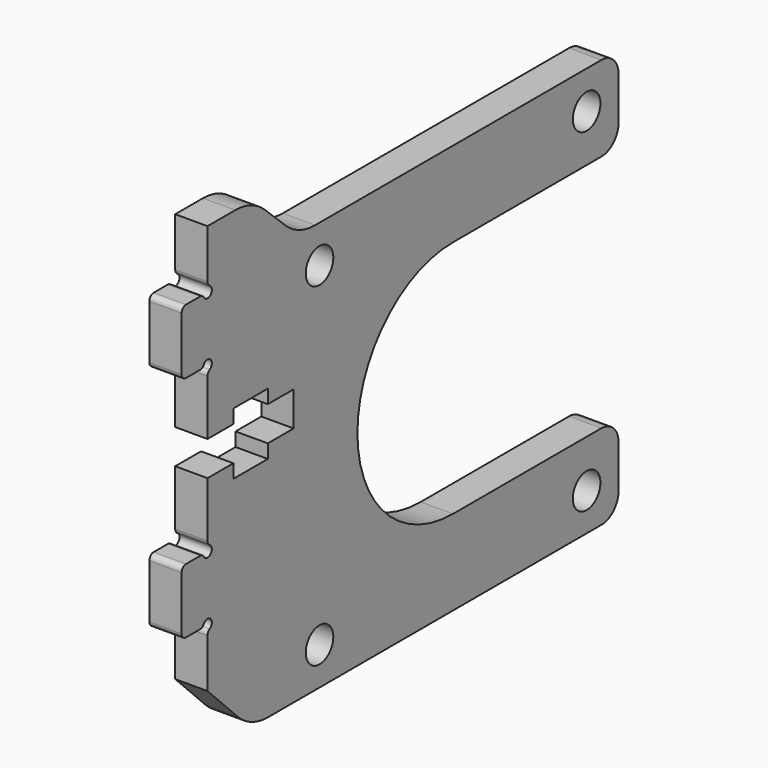
from build123d import *

# Parameters (mm, degrees)
F0_R     = 1.6
F1_DEPTH = 3


# Not quite as in the source:
# - ends of sketch curves that miss each other by under 0.0002 mm in the source are joined


with BuildPart() as f1:
    # F0 (on Right) → F1 (new body)
    with BuildSketch(Plane.YZ):
        with BuildLine():
            Line((6.490295, 24.126887), (6.490295, 20.926875))
            Line((6.490295, 20.926875), (3.490295, 20.926875))
            Line((3.490295, 20.926875), (3.490295, 19.651881))
            Line((3.490295, 19.651881), (-0.509733, 19.651881))
            Line((-0.509733, 19.651881), (-0.509733, 20.926875))
            Line((-0.509733, 20.926875), (-3.509705, 20.926875))
            Line((-3.509705, 20.926875), (-3.509702, 15.792903))
            ThreePointArc((-3.509702, 15.792903), (-3.4427150061, 15.542903527), (-3.2597030539, 15.3598909066))
            ThreePointArc((-3.2597030539, 15.3598909066), (-3.1561520924, 14.5733251264), (-3.9427177764, 14.6768791291))
            ThreePointArc((-3.9427177764, 14.6768791291), (-4.1257299355, 14.8598916646), (-4.37573, 14.926879))
            Line((-4.37573, 14.926879), (-6.009757, 14.926882))
            ThreePointArc((-6.009757, 14.926882), (-6.3633103906, 14.7804353906), (-6.509757, 14.426882))
            Line((-6.509757, 14.426882), (-6.509757, 9.426885))
            ThreePointArc((-6.509757, 9.426885), (-6.3633103906, 9.0733316094), (-6.009757, 8.926885))
            Line((-6.009757, 8.926885), (-4.375728, 8.926885))
            ThreePointArc((-4.375728, 8.926885), (-4.125728527, 8.9938719939), (-3.9427159066, 9.1768839461))
            ThreePointArc((-3.9427159066, 9.1768839461), (-3.1561511264, 9.2804349076), (-3.2597051291, 8.4938692236))
            ThreePointArc((-3.2597051291, 8.4938692236), (-3.4427176646, 8.3108560645), (-3.509705, 8.060856))
            Line((-3.509705, 8.060856), (-3.509702, 3.526887))
            Line((-3.509702, 3.526887), (0, 0))
            ThreePointArc((0, 0), (1.6251015018, -1.0901687381), (3.544158, -1.473111))
            Line((3.544158, -1.473111), (42.206461, -1.47311))
            ThreePointArc((42.206461, -1.47311), (43.6206745624, -0.8873235624), (44.206461, 0.52689))
            Line((44.206461, 0.52689), (44.206463, 4.426926))
            ThreePointArc((44.206463, 4.426926), (43.6206765624, 5.8411395624), (42.206463, 6.426926))
            Line((42.206463, 6.426926), (24.990243, 6.426926))
            ThreePointArc((24.990243, 6.426926), (13.890243, 17.526926), (24.990243, 28.626926))
            Line((24.990243, 28.626926), (42.206463, 28.626926))
            ThreePointArc((42.206463, 28.626926), (43.6206765624, 29.2127124376), (44.206463, 30.626926))
            Line((44.206463, 30.626926), (44.206463, 34.526876))
            ThreePointArc((44.206463, 34.526876), (43.6206745624, 35.9410875624), (42.206461, 36.526874))
            Line((42.206461, 36.526874), (8.985147, 36.526873))
            ThreePointArc((8.985147, 36.526873), (7.141367531, 36.8792416388), (5.5574640867, 37.8866820921))
            Line((5.5574640867, 37.8866820921), (3.135704, 40.167064))
            ThreePointArc((3.135704, 40.167064), (1.551800469, 41.1745043612), (-0.291979, 41.526873))
            Line((-0.291979, 41.526873), (-3.509705, 41.526873))
            Line((-3.509705, 41.526873), (-3.509702, 36.992904))
            ThreePointArc((-3.509702, 36.992904), (-3.4427150061, 36.742904527), (-3.2597030539, 36.5598919066))
            ThreePointArc((-3.2597030539, 36.5598919066), (-3.1561520924, 35.7733261264), (-3.9427177764, 35.8768801291))
            ThreePointArc((-3.9427177764, 35.8768801291), (-4.1257299355, 36.0598926646), (-4.37573, 36.12688))
            Line((-4.37573, 36.12688), (-6.009757, 36.126883))
            ThreePointArc((-6.009757, 36.126883), (-6.3633103906, 35.9804363906), (-6.509757, 35.626883))
            Line((-6.509757, 35.626883), (-6.509757, 30.626886))
            ThreePointArc((-6.509757, 30.626886), (-6.3633103906, 30.2733326094), (-6.009757, 30.126886))
            Line((-6.009757, 30.126886), (-4.375728, 30.126886))
            ThreePointArc((-4.375728, 30.126886), (-4.125728527, 30.1938729939), (-3.9427159066, 30.3768849461))
            ThreePointArc((-3.9427159066, 30.3768849461), (-3.1561511264, 30.4804359076), (-3.2597051291, 29.6938702236))
            ThreePointArc((-3.2597051291, 29.6938702236), (-3.4427176646, 29.5108580645), (-3.509705, 29.260858))
            Line((-3.509705, 29.260858), (-3.509705, 24.126887))
            Line((-3.509705, 24.126887), (-0.509733, 24.126887))
            Line((-0.509733, 24.126887), (-0.509733, 25.401881))
            Line((-0.509733, 25.401881), (3.490295, 25.401881))
            Line((3.490295, 25.401881), (3.490295, 24.126887))
            Line((3.490295, 24.126887), (6.490295, 24.126887))
        make_face()
        with Locations((9.490194, 2.026885)):
            Circle(F0_R, mode=Mode.SUBTRACT)
        with Locations((40.490194, 2.026885)):
            Circle(F0_R, mode=Mode.SUBTRACT)
        with Locations((9.490194, 33.026885)):
            Circle(F0_R, mode=Mode.SUBTRACT)
        with Locations((40.490194, 33.026885)):
            Circle(F0_R, mode=Mode.SUBTRACT)
    extrude(amount=F1_DEPTH)


solid = f1.part
